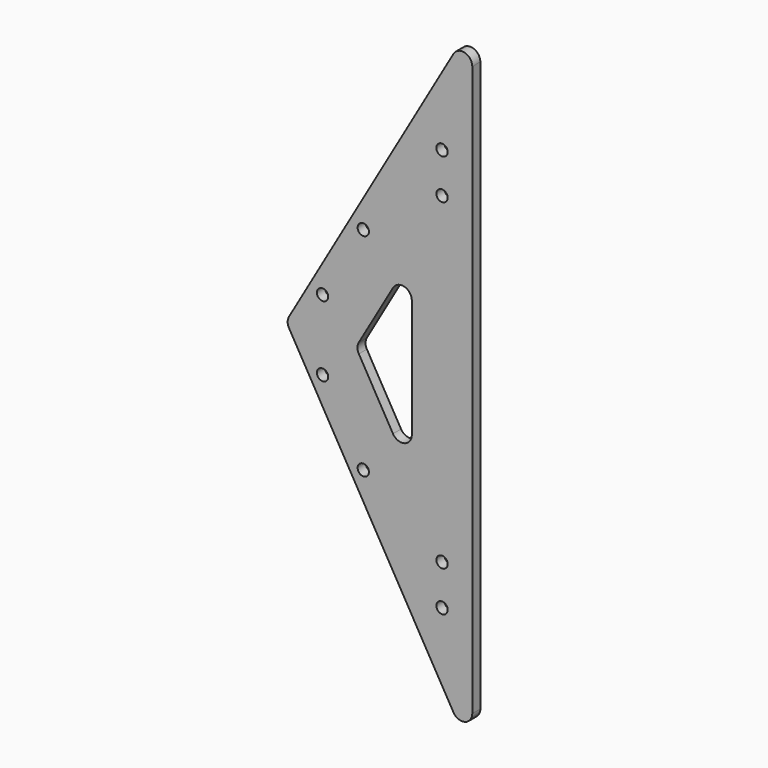
from build123d import *

# Parameters (mm, degrees)
F1_DEPTH = 6.35
F3_D     = 7.1374
F3_DEPTH = 304.8
F3_TIP   = 2.1442912911


# Not quite as in the source:
# - a feature names something its author has since deleted; it is built from what else it names


with BuildPart() as f1:
    # F0 (on Front) → F1 (new body)
    with BuildSketch(Plane.XZ):
        with BuildLine():
            ThreePointArc((-11.849261314, 20.5235226281), (-4.7064990636, 17.5648936311), (0, 23.6985226281))
            Line((0, 23.6985226281), (0, 382.7014773719))
            ThreePointArc((0, 382.7014773719), (-4.7064990636, 388.8351063689), (-11.849261314, 385.8764773719))
            Line((-11.849261314, 385.8764773719), (-115.4844875947, 206.375))
            ThreePointArc((-115.4844875947, 206.375), (-116.3352262806, 203.2), (-115.4844875947, 200.025))
            Line((-115.4844875947, 200.025), (-11.849261314, 20.5235226281))
        make_face()
        with BuildLine():
            ThreePointArc((-49.949261314, 243.6853416036), (-42.8064990636, 246.6439706005), (-38.1, 240.5103416036))
            Line((-38.1, 240.5103416036), (-38.1, 165.8896583964))
            ThreePointArc((-38.1, 165.8896583964), (-42.8064990636, 159.7560293995), (-49.949261314, 162.7146583964))
            Line((-49.949261314, 162.7146583964), (-71.4903970824, 200.025))
            ThreePointArc((-71.4903970824, 200.025), (-72.3411357684, 203.2), (-71.4903970824, 206.375))
            Line((-71.4903970824, 206.375), (-49.949261314, 243.6853416036))
        make_face(mode=Mode.SUBTRACT)
    extrude(amount=F1_DEPTH)

    # F3
    with Locations(Plane.XZ.offset(6.35)):
        with Locations((-94.3381810245, 225.425), (-94.3381810245, 180.975), (-19.05, 304.8), (-19.05, 101.6), (-19.05, 76.2), (-19.05, 330.2), (-68.674961559, 269.875), (-68.674961559, 136.525)):
            Hole(F3_D / 2, depth=F3_DEPTH)
            with Locations((0, 0, -(F3_DEPTH + F3_TIP / 2))):  # 118° drill point
                Cone(0, F3_D / 2, F3_TIP, mode=Mode.SUBTRACT)


solid = f1.part
